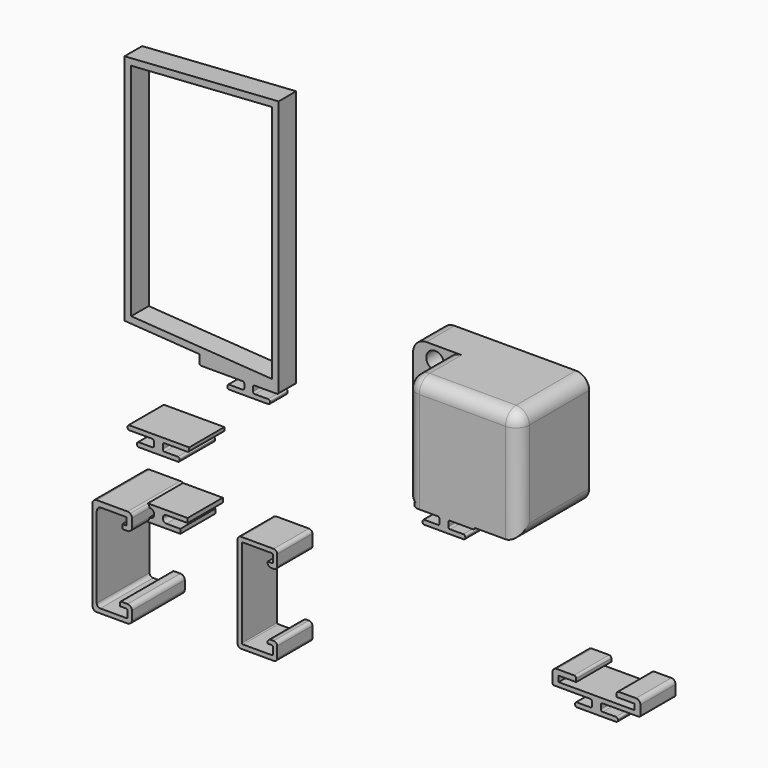
from build123d import *

# Parameters (mm, degrees)
F1_DEPTH      = 15
F0_W          = 0.5
F0_H          = 0.3
F2_DEPTH      = 10
F3_DEPTH      = 10
F4_DEPTH      = 10
F5_DEPTH      = 5
F6_DEPTH      = 20
F7_DEPTH      = 25
F8_DEPTH      = 10
F9_DEPTH      = 10
F10_R         = 2.05
F10_R_2       = 1.45
F10_R_3       = 1.1
F10_R_4       = 1
F10_R_5       = 0.75
F10_R_6       = 2
F10_R_7       = 2.5
F11_DEPTH     = 18
F12_W         = 12
F12_H         = 25
F13_DEPTH     = 8
F14_T1_DEPTH  = 24.5
F14_T3_DEPTH  = 23
F14_T5_DEPTH  = 9
F14_T7_DEPTH  = 35
F14_T9_DEPTH  = 19.0710678119
F14_T11_DEPTH = 29.5
F14_T13_DEPTH = 19.6
F14_T15_DEPTH = 30.1
F14_S19_W     = 3.06
F14_S19_H     = 3.06
F14_T20_DEPTH = 3.06
F14_S25_W     = 3.06
F14_S25_H     = 3.06
F14_T26_DEPTH = 3.06
F15_DEPTH     = 10


# Not quite as in the source:
# - a fillet or chamfer that OpenCascade refuses, or shapes differently, is made with other operations: its cross-section is extruded or revolved along the edge and cut away or added
# - a feature names something its author has since deleted; it is built from what else it names


with BuildPart() as f1:
    # F0 (on Front) → F1 (new body)
    with BuildSketch(Plane.XZ):
        Polygon((-3.2, 8), (-3.2, 8.3), (-3.3, 8.3), (-4.2, 8.3), (-4.2, 8), align=None)
        with BuildLine():
            Line((-6.6376544669, 11), (-6.6376544669, 10.2))
            Line((-6.6376544669, 10.2), (-4.5, 10.2))
            Line((-4.5, 10.2), (-3.3, 10.2))
            Line((-3.3, 10.2), (-2, 10.2))
            ThreePointArc((-2, 10.2), (-2.105572809, 10.6472135955), (-2.4, 11))
            Line((-2.4, 11), (-4.6376544669, 11))
            Line((-4.6376544669, 11), (-6.6376544669, 11))
        make_face()
        with BuildLine():
            Line((-10, -9), (-10, 9))
            Line((-10, 9), (-10, 9.4))
            ThreePointArc((-10, 9.4), (-9.7656854249, 9.9656854249), (-9.2, 10.2))
            Line((-9.2, 10.2), (-6.6376544669, 10.2))
            Line((-6.6376544669, 10.2), (-6.6376544669, 11))
            Line((-6.6376544669, 11), (-4.6376544669, 11))
            Line((-4.6376544669, 11), (-2.4, 11))
            ThreePointArc((-2.4, 11), (-2.683772234, 11.1486832981), (-3, 11.2))
            Line((-3, 11.2), (-10, 11.2))
            ThreePointArc((-10, 11.2), (-10.7071067812, 10.9071067812), (-11, 10.2))
            Line((-11, 10.2), (-11, -10.2))
            ThreePointArc((-11, -10.2), (-10.7071067812, -10.9071067812), (-10, -11.2))
            Line((-10, -11.2), (-3, -11.2))
            ThreePointArc((-3, -11.2), (-2.2928932188, -10.9071067812), (-2, -10.2))
            Line((-2, -10.2), (-2, -10))
            Line((-2, -10), (-2, -8.3))
            ThreePointArc((-2, -8.3), (-2.2928932188, -7.5928932188), (-3, -7.3))
            Line((-3, -7.3), (-4.4419462353, -7.3))
            ThreePointArc((-4.4419462353, -7.3), (-4.6540782697, -7.3878679656), (-4.7419462353, -7.6))
            Line((-4.7419462353, -7.6), (-4.7419462353, -8))
            Line((-4.7419462353, -8), (-3.2, -8))
            Line((-3.2, -8), (-3.2, -8.3171572875))
            ThreePointArc((-3.2, -8.3171572875), (-3.0550510257, -8.4267949192), (-3, -8.6))
            Line((-3, -8.6), (-3, -9.9))
            ThreePointArc((-3, -9.9), (-3.0878679656, -10.1121320344), (-3.3, -10.2))
            Line((-3.3, -10.2), (-9.2, -10.2))
            ThreePointArc((-9.2, -10.2), (-9.7656854249, -9.9656854249), (-10, -9.4))
            Line((-10, -9.4), (-10, -9))
        make_face()
        with BuildLine():
            ThreePointArc((-3, 8.6), (-3.0550510257, 8.4267949192), (-3.2, 8.3171572875))
            Line((-3.2, 8.3171572875), (-3.2, 8.3))
            Line((-3.2, 8.3), (-2, 8.3))
            Line((-2, 8.3), (-2, 10.2))
            Line((-2, 10.2), (-3.3, 10.2))
            ThreePointArc((-3.3, 10.2), (-3.0878679656, 10.1121320344), (-3, 9.9))
            Line((-3, 9.9), (-3, 8.6))
        make_face()
        with BuildLine():
            Line((-2, 8.3), (-3.2, 8.3))
            Line((-3.2, 8.3), (-3.2, 8))
            Line((-3.2, 8), (-3.2, 7.3))
            Line((-3.2, 7.3), (-3, 7.3))
            ThreePointArc((-3, 7.3), (-2.2928932188, 7.5928932188), (-2, 8.3))
        make_face()
        with BuildLine():
            Line((-3.2, 7.3), (-3.2, 8))
            Line((-3.2, 8), (-4.2, 8))
            Line((-4.2, 8), (-4.2, 7.6))
            ThreePointArc((-4.2, 7.6), (-4.1121320344, 7.3878679656), (-3.9, 7.3))
            Line((-3.9, 7.3), (-3.2, 7.3))
        make_face()
        with BuildLine():
            ThreePointArc((-10, 9), (-9.7071067812, 9.7071067812), (-9, 10))
            Line((-9, 10), (-3.2, 10))
            Line((-3.2, 10), (-3.2, 8.8017444491))
            Line((-3.2, 8.8017444491), (-3.2, 8.3171572875))
            ThreePointArc((-3.2, 8.3171572875), (-3.0550510257, 8.4267949192), (-3, 8.6))
            Line((-3, 8.6), (-3, 9.9))
            ThreePointArc((-3, 9.9), (-3.0878679656, 10.1121320344), (-3.3, 10.2))
            Line((-3.3, 10.2), (-4.5, 10.2))
            Line((-4.5, 10.2), (-6.6376544669, 10.2))
            Line((-6.6376544669, 10.2), (-9.2, 10.2))
            ThreePointArc((-9.2, 10.2), (-9.7656854249, 9.9656854249), (-10, 9.4))
            Line((-10, 9.4), (-10, 9))
        make_face()
        with BuildLine():
            ThreePointArc((-3.3, -8.3), (-3.2492694064, -8.3043204321), (-3.2, -8.3171572875))
            Line((-3.2, -8.3171572875), (-3.2, -8))
            Line((-3.2, -8), (-4.7419462353, -8))
            Line((-4.7419462353, -8), (-4.7419462353, -8.3))
            Line((-4.7419462353, -8.3), (-3.3, -8.3))
        make_face()
    extrude(amount=F1_DEPTH)


with BuildPart() as f2:
    # F0 (on Front) → F2 (new body)
    with BuildSketch(Plane.XZ):
        with BuildLine():
            Line((-2, 8.3), (-3.2, 8.3))
            Line((-3.2, 8.3), (-3.2, 8))
            Line((-3.2, 8), (-3.2, 7.3))
            Line((-3.2, 7.3), (-3, 7.3))
            ThreePointArc((-3, 7.3), (-2.2928932188, 7.5928932188), (-2, 8.3))
        make_face()
        Polygon((-3.2, 8), (-3.2, 8.3), (-3.3, 8.3), (-4.2, 8.3), (-4.2, 8), align=None)
        with BuildLine():
            Line((-6.6376544669, 11), (-6.6376544669, 10.2))
            Line((-6.6376544669, 10.2), (-4.5, 10.2))
            Line((-4.5, 10.2), (-3.3, 10.2))
            Line((-3.3, 10.2), (-2, 10.2))
            ThreePointArc((-2, 10.2), (-2.105572809, 10.6472135955), (-2.4, 11))
            Line((-2.4, 11), (-4.6376544669, 11))
            Line((-4.6376544669, 11), (-6.6376544669, 11))
        make_face()
        with BuildLine():
            Line((-3.2, 7.3), (-3.2, 8))
            Line((-3.2, 8), (-4.2, 8))
            Line((-4.2, 8), (-4.2, 7.6))
            ThreePointArc((-4.2, 7.6), (-4.1121320344, 7.3878679656), (-3.9, 7.3))
            Line((-3.9, 7.3), (-3.2, 7.3))
        make_face()
        with BuildLine():
            Line((-1.7984359711, 8.3), (-2, 8.3))
            ThreePointArc((-2, 8.3), (-2.2928932188, 7.5928932188), (-3, 7.3))
            Line((-3, 7.3), (-2, 7.3))
            Line((-2, 7.3), (5, 7.3))
            Line((5, 7.3), (5, 8))
            Line((5, 8), (3.2, 8))
            Line((3.2, 8), (3.2, 8.3))
            Line((3.2, 8.3), (1.7984359711, 8.3))
            ThreePointArc((1.7984359711, 8.3), (1.2153407816, 8.5522774425), (1, 9.15))
            Line((1, 9.15), (1, 9.2))
            ThreePointArc((1, 9.2), (1.2343145751, 9.7656854249), (1.8, 10))
            Line((1.8, 10), (3.2, 10))
            Line((3.2, 10), (6.6376544669, 10))
            Line((6.6376544669, 10), (6.6376544669, 11))
            Line((6.6376544669, 11), (4.5, 11))
            Line((4.5, 11), (-2.4, 11))
            ThreePointArc((-2.4, 11), (-2.105572809, 10.6472135955), (-2, 10.2))
            Line((-2, 10.2), (-1.8, 10.2))
            ThreePointArc((-1.8, 10.2), (-1.2343145751, 9.9656854249), (-1, 9.4))
            Line((-1, 9.4), (-1, 9.15))
            ThreePointArc((-1, 9.15), (-1.2153407816, 8.5522774425), (-1.7984359711, 8.3))
        make_face()
        with Locations((-4.45, 8.15)):
            Rectangle(F0_W, F0_H)
        Polygon((-4.2, 7.6), (-4.2, 8), (-4.7, 8), (-4.7, 7.3), (-4.2, 7.3), align=None)
        with BuildLine():
            ThreePointArc((-3.9, 7.3), (-4.1121320344, 7.3878679656), (-4.2, 7.6))
            Line((-4.2, 7.6), (-4.2, 7.3))
            Line((-4.2, 7.3), (-3.9, 7.3))
        make_face()
        Polygon((3.2, 8), (5, 8), (5, 8.3), (4.5, 8.3), (3.2, 8.3), align=None)
    extrude(amount=F2_DEPTH)


with BuildPart() as f3:
    # F0 (on Front) → F3 (new body)
    with BuildSketch(Plane.XZ):
        with BuildLine():
            Line((25.8, 8.2), (24.8, 8.2))
            Line((24.8, 8.2), (24.8, 8))
            ThreePointArc((24.8, 8), (25.0343145751, 7.4343145751), (25.6, 7.2))
            Line((25.6, 7.2), (26.2, 7.2))
            ThreePointArc((26.2, 7.2), (26.7656854249, 7.4343145751), (27, 8))
            Line((27, 8), (27, 10.4))
            ThreePointArc((27, 10.4), (26.7656854249, 10.9656854249), (26.2, 11.2))
            Line((26.2, 11.2), (18.8, 11.2))
            ThreePointArc((18.8, 11.2), (18.2343145751, 10.9656854249), (18, 10.4))
            Line((18, 10.4), (18, -10.4))
            ThreePointArc((18, -10.4), (18.2343145751, -10.9656854249), (18.8, -11.2))
            Line((18.8, -11.2), (26.2, -11.2))
            ThreePointArc((26.2, -11.2), (26.7656854249, -10.9656854249), (27, -10.4))
            Line((27, -10.4), (27, -8))
            ThreePointArc((27, -8), (26.7656854249, -7.4343145751), (26.2, -7.2))
            Line((26.2, -7.2), (25.6, -7.2))
            ThreePointArc((25.6, -7.2), (25.0343145751, -7.4343145751), (24.8, -8))
            Line((24.8, -8), (24.8, -8.2))
            Line((24.8, -8.2), (25.8, -8.2))
            ThreePointArc((25.8, -8.2), (25.9414213562, -8.2585786438), (26, -8.4))
            Line((26, -8.4), (26, -10))
            ThreePointArc((26, -10), (25.9414213562, -10.1414213562), (25.8, -10.2))
            Line((25.8, -10.2), (19.2, -10.2))
            ThreePointArc((19.2, -10.2), (19.0585786438, -10.1414213562), (19, -10))
            Line((19, -10), (19, 10))
            ThreePointArc((19, 10), (19.0585786438, 10.1414213562), (19.2, 10.2))
            Line((19.2, 10.2), (25.8, 10.2))
            ThreePointArc((25.8, 10.2), (25.9414213562, 10.1414213562), (26, 10))
            Line((26, 10), (26, 8.4))
            ThreePointArc((26, 8.4), (25.9414213562, 8.2585786438), (25.8, 8.2))
        make_face()
    extrude(amount=F3_DEPTH)


with BuildPart() as f4:
    # F0 (on Front) → F4 (new body)
    with BuildSketch(Plane.XZ):
        with BuildLine():
            Line((7, 25.2431258559), (-6.6, 25.2431258559))
            ThreePointArc((-6.6, 25.2431258559), (-6.8828427125, 25.1259685684), (-7, 24.8431258559))
            Line((-7, 24.8431258559), (-7, 24.6431258559))
            ThreePointArc((-7, 24.6431258559), (-6.8828427125, 24.3602831434), (-6.6, 24.2431258559))
            Line((-6.6, 24.2431258559), (-1.4, 24.2431258559))
            ThreePointArc((-1.4, 24.2431258559), (-1.1171572875, 24.1259685684), (-1, 23.8431258559))
            Line((-1, 23.8431258559), (-1, 22.9431258559))
            ThreePointArc((-1, 22.9431258559), (-1.1171572875, 22.6602831434), (-1.4, 22.5431258559))
            Line((-1.4, 22.5431258559), (-4.45, 22.5431258559))
            ThreePointArc((-4.45, 22.5431258559), (-4.7328427125, 22.4259685684), (-4.85, 22.1431258559))
            Line((-4.85, 22.1431258559), (-4.85, 21.9431258559))
            ThreePointArc((-4.85, 21.9431258559), (-4.7328427125, 21.6602831434), (-4.45, 21.5431258559))
            Line((-4.45, 21.5431258559), (4.45, 21.5431258559))
            ThreePointArc((4.45, 21.5431258559), (4.7328427125, 21.6602831434), (4.85, 21.9431258559))
            Line((4.85, 21.9431258559), (4.85, 22.1431258559))
            ThreePointArc((4.85, 22.1431258559), (4.7328427125, 22.4259685684), (4.45, 22.5431258559))
            Line((4.45, 22.5431258559), (1.4, 22.5431258559))
            ThreePointArc((1.4, 22.5431258559), (1.1171572875, 22.6602831434), (1, 22.9431258559))
            Line((1, 22.9431258559), (1, 23.8431258559))
            ThreePointArc((1, 23.8431258559), (1.1171572875, 24.1259685684), (1.4, 24.2431258559))
            Line((1.4, 24.2431258559), (6.6, 24.2431258559))
            ThreePointArc((6.6, 24.2431258559), (6.8828427125, 24.3602831434), (7, 24.6431258559))
            Line((7, 24.6431258559), (7, 25.2431258559))
        make_face()
    extrude(amount=F4_DEPTH)


with BuildPart() as f5:
    # F0 (on Front) → F5 (new body)
    with BuildSketch(Plane.XZ):
        with BuildLine():
            Line((-11.6821215733, 95.3670967946), (-11.6821215733, 42.4618956788))
            Line((-11.6821215733, 42.4618956788), (5.3178784267, 41.3197081788))
            Line((5.3178784267, 41.3197081788), (5.3178784267, 39.7103331788))
            Line((5.3178784267, 39.7103331788), (5.3178784267, 39.5103331788))
            ThreePointArc((5.3178784267, 39.5103331788), (5.4350357142, 39.2274904663), (5.7178784267, 39.1103331788))
            Line((5.7178784267, 39.1103331788), (15.1178784267, 39.1103331788))
            ThreePointArc((15.1178784267, 39.1103331788), (15.4007211391, 38.9931758913), (15.5178784267, 38.7103331788))
            Line((15.5178784267, 38.7103331788), (15.5178784267, 37.8103331788))
            ThreePointArc((15.5178784267, 37.8103331788), (15.4007211391, 37.5274904663), (15.1178784267, 37.4103331788))
            Line((15.1178784267, 37.4103331788), (12.0678784267, 37.4103331788))
            ThreePointArc((12.0678784267, 37.4103331788), (11.7850357142, 37.2931758913), (11.6678784267, 37.0103331788))
            Line((11.6678784267, 37.0103331788), (11.6678784267, 36.8103331788))
            ThreePointArc((11.6678784267, 36.8103331788), (11.7850357142, 36.5274904663), (12.0678784267, 36.4103331788))
            Line((12.0678784267, 36.4103331788), (20.9678784267, 36.4103331788))
            ThreePointArc((20.9678784267, 36.4103331788), (21.2507211391, 36.5274904663), (21.3678784267, 36.8103331788))
            Line((21.3678784267, 36.8103331788), (21.3678784267, 37.0103331788))
            ThreePointArc((21.3678784267, 37.0103331788), (21.2507211391, 37.2931758913), (20.9678784267, 37.4103331788))
            Line((20.9678784267, 37.4103331788), (17.9178784267, 37.4103331788))
            ThreePointArc((17.9178784267, 37.4103331788), (17.6350357142, 37.5274904663), (17.5178784267, 37.8103331788))
            Line((17.5178784267, 37.8103331788), (17.5178784267, 38.7103331788))
            ThreePointArc((17.5178784267, 38.7103331788), (17.6350357142, 38.9931758913), (17.9178784267, 39.1103331788))
            Line((17.9178784267, 39.1103331788), (22.9178784267, 39.1103331788))
            ThreePointArc((22.9178784267, 39.1103331788), (23.2007211391, 39.2274904663), (23.3178784267, 39.5103331788))
            Line((23.3178784267, 39.5103331788), (23.3178784267, 40.1103331788))
            Line((23.3178784267, 40.1103331788), (23.3178784267, 97.7186592946))
            Line((23.3178784267, 97.7186592946), (-11.6821215733, 95.3670967946))
        make_face()
        Polygon((-10.1821215733, 93.9644962367), (21.8178784267, 96.1144962367), (21.8178784267, 41.7144962367), (-10.1821215733, 43.8644962367), align=None, mode=Mode.SUBTRACT)
    extrude(amount=F5_DEPTH)


with BuildPart() as f6:
    # F0 (on Front) → F6 (new body)
    with BuildSketch(Plane.XZ):
        with BuildLine():
            Line((79.8733060375, 37.5043063505), (66.2733060375, 37.5043063505))
            ThreePointArc((66.2733060375, 37.5043063505), (65.9904633251, 37.387149063), (65.8733060375, 37.1043063505))
            Line((65.8733060375, 37.1043063505), (65.8733060375, 36.9043063505))
            ThreePointArc((65.8733060375, 36.9043063505), (65.9904633251, 36.621463638), (66.2733060375, 36.5043063505))
            Line((66.2733060375, 36.5043063505), (71.4733060375, 36.5043063505))
            ThreePointArc((71.4733060375, 36.5043063505), (71.75614875, 36.387149063), (71.8733060375, 36.1043063505))
            Line((71.8733060375, 36.1043063505), (71.8733060375, 35.2043063505))
            ThreePointArc((71.8733060375, 35.2043063505), (71.75614875, 34.921463638), (71.4733060375, 34.8043063505))
            Line((71.4733060375, 34.8043063505), (68.4233060375, 34.8043063505))
            ThreePointArc((68.4233060375, 34.8043063505), (68.1404633251, 34.687149063), (68.0233060375, 34.4043063505))
            Line((68.0233060375, 34.4043063505), (68.0233060375, 34.2043063505))
            ThreePointArc((68.0233060375, 34.2043063505), (68.1404633251, 33.921463638), (68.4233060375, 33.8043063505))
            Line((68.4233060375, 33.8043063505), (77.3233060375, 33.8043063505))
            ThreePointArc((77.3233060375, 33.8043063505), (77.60614875, 33.921463638), (77.7233060375, 34.2043063505))
            Line((77.7233060375, 34.2043063505), (77.7233060375, 34.4043063505))
            ThreePointArc((77.7233060375, 34.4043063505), (77.60614875, 34.687149063), (77.3233060375, 34.8043063505))
            Line((77.3233060375, 34.8043063505), (74.2733060375, 34.8043063505))
            ThreePointArc((74.2733060375, 34.8043063505), (73.9904633251, 34.921463638), (73.8733060375, 35.2043063505))
            Line((73.8733060375, 35.2043063505), (73.8733060375, 36.1043063505))
            ThreePointArc((73.8733060375, 36.1043063505), (73.9904633251, 36.387149063), (74.2733060375, 36.5043063505))
            Line((74.2733060375, 36.5043063505), (79.4733060375, 36.5043063505))
            ThreePointArc((79.4733060375, 36.5043063505), (79.75614875, 36.621463638), (79.8733060375, 36.9043063505))
            Line((79.8733060375, 36.9043063505), (79.8733060375, 37.5043063505))
        make_face()
    extrude(amount=F6_DEPTH)

    # F7 (add): a face of the model
    f7_faces = [f6.faces().sort_by_distance(p)[0] for p in [
        (73.0733060375, -10, 37.5043063505),
    ]]
    extrude(f7_faces, amount=F7_DEPTH)

    # F8 (add): a face of the model
    f8_faces = [f6.faces().sort_by_distance(p)[0] for p in [
        (79.8733060375, -10, 49.7043063505),
    ]]
    extrude(f8_faces, amount=F8_DEPTH)

    # F9 (add): a face of the model
    f9_faces = [f6.faces().sort_by_distance(p)[0] for p in [
        (66.2733060375, -10, 50.0043063505),
    ]]
    extrude(f9_faces, amount=F9_DEPTH)

    # F10 (on face) → F11 (cut, through all)
    with BuildSketch(Plane(origin=(0, 0, 0), x_dir=(-1, 0, 0), z_dir=(0, 1, 0))):
        with BuildLine():
            Line((-86.4733060375, 47.5043063505), (-68.2733060375, 47.5043063505))
            ThreePointArc((-68.2733060375, 47.5043063505), (-66.8590924752, 48.0900927881), (-66.2733060375, 49.5043063505))
            Line((-66.2733060375, 49.5043063505), (-66.2733060375, 59.3043063505))
            ThreePointArc((-66.2733060375, 59.3043063505), (-66.8590924752, 60.7185199129), (-68.2733060375, 61.3043063505))
            Line((-68.2733060375, 61.3043063505), (-86.4733060375, 61.3043063505))
            ThreePointArc((-86.4733060375, 61.3043063505), (-87.8875195999, 60.7185199129), (-88.4733060375, 59.3043063505))
            Line((-88.4733060375, 59.3043063505), (-88.4733060375, 49.5043063505))
            ThreePointArc((-88.4733060375, 49.5043063505), (-87.8875195999, 48.0900927881), (-86.4733060375, 47.5043063505))
        make_face()
        with Locations((-61.2733060375, 40.7543063505)):
            Circle(F10_R)
        with Locations((-61.2733060375, 45.4543063505)):
            Circle(F10_R_2)
        with Locations((-61.2733060375, 49.2043063505)):
            Circle(F10_R_3)
        with Locations((-61.2733060375, 52.5043063505)):
            Circle(F10_R_4)
        with Locations((-61.2733060375, 55.4543063505)):
            Circle(F10_R_5)
        with Locations((-61.2733060375, 59.4043063505)):
            Circle(F10_R_6)
        with Locations((-86.1733060375, 41.9043063505)):
            Circle(F10_R_7)
        with Locations((-79.9733060375, 41.9043063505)):
            Circle(F10_R_7)
        with Locations((-73.7733060375, 41.9043063505)):
            Circle(F10_R_7)
        with Locations((-67.5733060375, 41.9043063505)):
            Circle(F10_R_7)
    extrude(amount=-F11_DEPTH, mode=Mode.SUBTRACT)

    # F12 (on face) → F13 (cut)
    with BuildSketch(Plane(origin=(56.2733060375, 0, 0), x_dir=(0, -1, 0), z_dir=(-1, 0, 0))):
        with Locations((14, 50.0043063505)):
            Rectangle(F12_W, F12_H)
    extrude(amount=-F13_DEPTH, mode=Mode.SUBTRACT)

    # F14: fillet of radius 3 on 9 edges, made by hand

    # F14_s2 → F14_t1 (cut)
    with BuildSketch(Plane.XZ.offset(-7.5)):
        with BuildLine():
            ThreePointArc((86.8733060375, 62.5043063505), (88.9946263811, 61.6256266941), (89.8733060375, 59.5043063505))
            Line((89.8733060375, 59.5043063505), (89.8733060375, 62.5043063505))
            Line((89.8733060375, 62.5043063505), (86.8733060375, 62.5043063505))
        make_face()
    extrude(amount=F14_T1_DEPTH, mode=Mode.SUBTRACT)

    # F14_s4 → F14_t3 (cut)
    with BuildSketch(Plane.XZ.offset(-7.5)):
        with BuildLine():
            ThreePointArc((56.2733060375, 59.5043063505), (57.151985694, 61.6256266941), (59.2733060375, 62.5043063505))
            Line((59.2733060375, 62.5043063505), (56.2733060375, 62.5043063505))
            Line((56.2733060375, 62.5043063505), (56.2733060375, 59.5043063505))
        make_face()
        with BuildLine():
            ThreePointArc((59.2733060375, 37.5043063505), (57.151985694, 38.382986007), (56.2733060375, 40.5043063505))
            Line((56.2733060375, 40.5043063505), (56.2733060375, 37.5043063505))
            Line((56.2733060375, 37.5043063505), (59.2733060375, 37.5043063505))
        make_face()
    extrude(amount=F14_T3_DEPTH, mode=Mode.SUBTRACT)

    # F14_s6 → F14_t5 (cut)
    with BuildSketch(Plane.XZ.offset(8)):
        with BuildLine():
            ThreePointArc((64.2733060375, 59.5043063505), (65.151985694, 61.6256266941), (67.2733060375, 62.5043063505))
            Line((67.2733060375, 62.5043063505), (64.2733060375, 62.5043063505))
            Line((64.2733060375, 62.5043063505), (64.2733060375, 59.5043063505))
        make_face()
    extrude(amount=F14_T5_DEPTH, mode=Mode.SUBTRACT)

    # F14_s8 → F14_t7 (cut)
    with BuildSketch(Plane.XZ.offset(-7.5)):
        with BuildLine():
            ThreePointArc((89.8733060375, 39.9043063505), (88.9946263811, 37.782986007), (86.8733060375, 36.9043063505))
            Line((86.8733060375, 36.9043063505), (89.8733060375, 36.9043063505))
            Line((89.8733060375, 36.9043063505), (89.8733060375, 39.9043063505))
        make_face()
    extrude(amount=F14_T7_DEPTH, mode=Mode.SUBTRACT)

    # F14_s10 → F14_t9 (cut)
    with BuildSketch(Plane.XZ.offset(8)):
        with BuildLine():
            ThreePointArc((66.2733060375, 37.5043063505), (64.8238162947, 38.6006826677), (64.2733060375, 40.3327334753))
            Line((64.2733060375, 40.3327334753), (64.2733060375, 37.5043063505))
            Line((64.2733060375, 37.5043063505), (66.2733060375, 37.5043063505))
        make_face()
    extrude(amount=F14_T9_DEPTH, mode=Mode.SUBTRACT)

    # F14_s12 → F14_t11 (cut)
    with BuildSketch(Plane.XY.offset(30.0043063505)):
        with BuildLine():
            ThreePointArc((67.2733060375, -20), (65.151985694, -19.1213203436), (64.2733060375, -17))
            Line((64.2733060375, -17), (64.2733060375, -20))
            Line((64.2733060375, -20), (67.2733060375, -20))
        make_face()
    extrude(amount=F14_T11_DEPTH, mode=Mode.SUBTRACT)

    # F14_s14 → F14_t13 (cut)
    with BuildSketch(Plane.YZ.offset(67.2733060375)):
        with BuildLine():
            ThreePointArc((-20, 59.5043063505), (-19.1213203436, 61.6256266941), (-17, 62.5043063505))
            Line((-17, 62.5043063505), (-20, 62.5043063505))
            Line((-20, 62.5043063505), (-20, 59.5043063505))
        make_face()
    extrude(amount=F14_T13_DEPTH, mode=Mode.SUBTRACT)

    # F14_s16 → F14_t15 (cut)
    with BuildSketch(Plane.XY.offset(29.4043063505)):
        with BuildLine():
            ThreePointArc((86.8733060375, -20), (88.9946263811, -19.1213203436), (89.8733060375, -17))
            Line((89.8733060375, -17), (89.8733060375, -20))
            Line((89.8733060375, -20), (86.8733060375, -20))
        make_face()
    extrude(amount=F14_T15_DEPTH, mode=Mode.SUBTRACT)


with BuildPart() as f14_tool18:
    # F14_s19 → F14_t20 (new body)
    with BuildSketch(Plane.XY.offset(59.5043063505)):
        with Locations((88.4033060375, -18.53)):
            Rectangle(F14_S19_W, F14_S19_H)
    extrude(amount=F14_T20_DEPTH)

    # F14_s21 → F14_t22 (revolve, cut)
    with BuildSketch(Plane(origin=(86.8733060375, -17, 59.5043063505), x_dir=(-0.7071067812, 0.7071067812, 0), z_dir=(0.7071067812, 0.7071067812, 0))):
        with BuildLine():
            ThreePointArc((0, -3), (3, 0), (0, 3))
            Line((0, 3), (0, -3))
        make_face()
    revolve(axis=Axis((86.8733060375, -17, 59.5043063505), (0, 0, 1)), mode=Mode.SUBTRACT)


with BuildPart() as f6_1:
    add(f6.part)

    # F14_t17: cut F14_tool18
    add(f14_tool18.part, mode=Mode.SUBTRACT)


with BuildPart() as f14_tool24:
    # F14_s25 → F14_t26 (new body)
    with BuildSketch(Plane.XY.offset(59.5043063505)):
        with Locations((65.7433060375, -18.53)):
            Rectangle(F14_S25_W, F14_S25_H)
    extrude(amount=F14_T26_DEPTH)

    # F14_s27 → F14_t28 (revolve, cut)
    with BuildSketch(Plane(origin=(67.2733060375, -17, 59.5043063505), x_dir=(0.7071067812, 0.7071067812, 0), z_dir=(0.7071067812, -0.7071067812, 0))):
        with BuildLine():
            ThreePointArc((0, -3), (3, 0), (0, 3))
            Line((0, 3), (0, -3))
        make_face()
    revolve(axis=Axis((67.2733060375, -17, 59.5043063505), (0, 0, 1)), mode=Mode.SUBTRACT)


with BuildPart() as f6_2:
    add(f6_1.part)

    # F14_t23: cut F14_tool24
    add(f14_tool24.part, mode=Mode.SUBTRACT)


with BuildPart() as f15:
    # F0 (on Front) → F15 (new body)
    with BuildSketch(Plane.XZ):
        with BuildLine():
            Line((90.9252945752, 5.5927135982), (89.5252945752, 5.5927135982))
            Line((89.5252945752, 5.5927135982), (89.5252945752, 5.1751870386))
            Line((89.5252945752, 5.1751870386), (89.5252945752, 4.9927135982))
            ThreePointArc((89.5252945752, 4.9927135982), (89.6424518627, 4.7098708857), (89.9252945752, 4.5927135982))
            Line((89.9252945752, 4.5927135982), (98.1252945752, 4.5927135982))
            ThreePointArc((98.1252945752, 4.5927135982), (98.4081372876, 4.4755563106), (98.5252945752, 4.1927135982))
            Line((98.5252945752, 4.1927135982), (98.5252945752, 3.2927135982))
            ThreePointArc((98.5252945752, 3.2927135982), (98.4081372876, 3.0098708857), (98.1252945752, 2.8927135982))
            Line((98.1252945752, 2.8927135982), (95.0752945752, 2.8927135982))
            ThreePointArc((95.0752945752, 2.8927135982), (94.7924518627, 2.7755563106), (94.6752945752, 2.4927135982))
            Line((94.6752945752, 2.4927135982), (94.6752945752, 2.2927135982))
            ThreePointArc((94.6752945752, 2.2927135982), (94.7924518627, 2.0098708857), (95.0752945752, 1.8927135982))
            Line((95.0752945752, 1.8927135982), (103.9752945752, 1.8927135982))
            ThreePointArc((103.9752945752, 1.8927135982), (104.2581372876, 2.0098708857), (104.3752945752, 2.2927135982))
            Line((104.3752945752, 2.2927135982), (104.3752945752, 2.4927135982))
            ThreePointArc((104.3752945752, 2.4927135982), (104.2581372876, 2.7755563106), (103.9752945752, 2.8927135982))
            Line((103.9752945752, 2.8927135982), (100.9252945752, 2.8927135982))
            ThreePointArc((100.9252945752, 2.8927135982), (100.6424518627, 3.0098708857), (100.5252945752, 3.2927135982))
            Line((100.5252945752, 3.2927135982), (100.5252945752, 4.1927135982))
            ThreePointArc((100.5252945752, 4.1927135982), (100.6424518627, 4.4755563106), (100.9252945752, 4.5927135982))
            Line((100.9252945752, 4.5927135982), (109.1252945752, 4.5927135982))
            ThreePointArc((109.1252945752, 4.5927135982), (109.4081372876, 4.7098708857), (109.5252945752, 4.9927135982))
            Line((109.5252945752, 4.9927135982), (109.5252945752, 5.5927135982))
            Line((109.5252945752, 5.5927135982), (108.1252945752, 5.5927135982))
            Line((108.1252945752, 5.5927135982), (90.9252945752, 5.5927135982))
        make_face()
        with BuildLine():
            Line((108.1252945752, 6.8927135982), (108.1252945752, 5.5927135982))
            Line((108.1252945752, 5.5927135982), (109.5252945752, 5.5927135982))
            Line((109.5252945752, 5.5927135982), (109.5252945752, 7.0927135982))
            ThreePointArc((109.5252945752, 7.0927135982), (109.2324013564, 7.7998203793), (108.5252945752, 8.0927135982))
            Line((108.5252945752, 8.0927135982), (104.6252945752, 8.0927135982))
            ThreePointArc((104.6252945752, 8.0927135982), (104.2717411846, 7.9462669888), (104.1252945752, 7.5927135982))
            Line((104.1252945752, 7.5927135982), (104.1252945752, 6.8927135982))
            Line((104.1252945752, 6.8927135982), (108.1252945752, 6.8927135982))
        make_face()
        with BuildLine():
            Line((89.5252945752, 7.0927135982), (89.5252945752, 5.5927135982))
            Line((89.5252945752, 5.5927135982), (90.9252945752, 5.5927135982))
            Line((90.9252945752, 5.5927135982), (90.9252945752, 6.8927135982))
            Line((90.9252945752, 6.8927135982), (94.9252945752, 6.8927135982))
            Line((94.9252945752, 6.8927135982), (94.9252945752, 7.5927135982))
            ThreePointArc((94.9252945752, 7.5927135982), (94.7788479658, 7.9462669888), (94.4252945752, 8.0927135982))
            Line((94.4252945752, 8.0927135982), (90.5252945752, 8.0927135982))
            ThreePointArc((90.5252945752, 8.0927135982), (89.818187794, 7.7998203793), (89.5252945752, 7.0927135982))
        make_face()
    extrude(amount=F15_DEPTH)


solid = Compound([f1.part, f2.part, f3.part, f4.part, f5.part, f6_2.part, f15.part])
